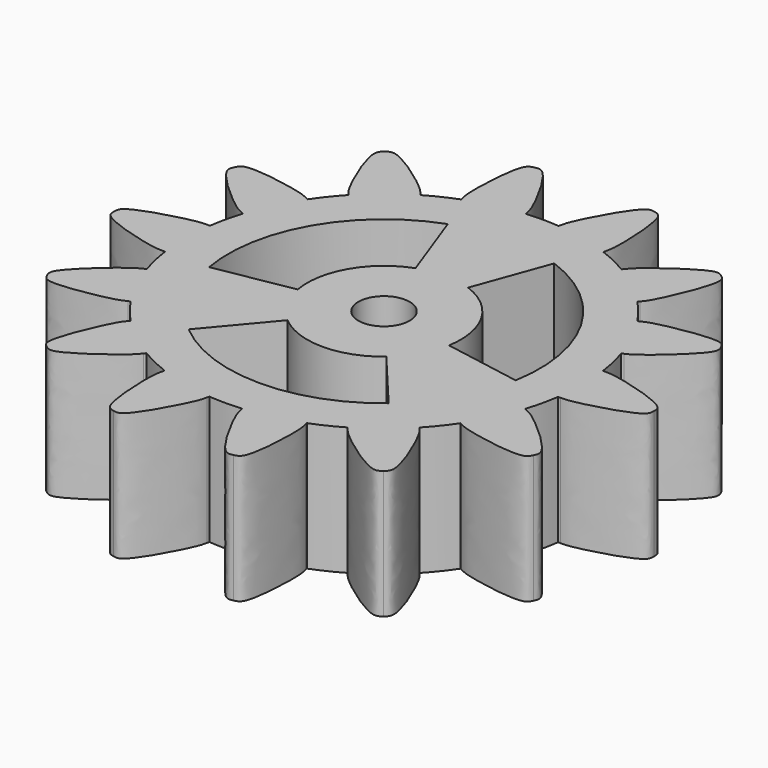
from build123d import *

# Parameters (mm, degrees)
F0_R     = 5.3351790251
F1_DEPTH = 10
F2_DEPTH = 10
F3_COUNT = 14
F4_R     = 15.5
F5_DEPTH = 10
F8_DEPTH = 10
F7_R     = 2
F9_DEPTH = 10


# Not quite as in the source:
# - a feature names something its author has since deleted; it is built from what else it names


with BuildPart() as f1:
    # F0 (on Top) → F1 (new body)
    with BuildSketch(Plane.XY):
        Circle(F0_R)
    extrude(amount=F1_DEPTH)



with BuildPart() as f2:
    # F0 (on Top) → F2 (new body)
    with BuildSketch(Plane.XY):
        with BuildLine():
            Line((-21.0813645951, 0), (-15.5169374102, 0))
            Line((-15.5169374102, 0), (-15.5169374102, 2.1929510403))
            add(Edge.make_bspline(
                [(-15.5169374102, 2.1929510403), (-15.7431787684, 2.1963284468), (-16.4584927159, 2.2070069607), (-21.1021855068, 0.9410331304), (-21.0859014535, 0.2050513008), (-21.0813645951, 0)],
                knots=[0, 0, 0, 0, 0.2502118821, 0.7911020914, 1, 1, 1, 1], degree=3))
        make_face()
        Polygon((-15.5169374102, -2.1929510403), (-13.8607590251, -2.1929510403), (-13.8607590251, 2.1929510403), (-15.5169374102, 2.1929510403), (-15.5169374102, 0), align=None)
        with BuildLine():
            add(Edge.make_bspline(
                [(-15.5169374102, -2.1929510403), (-15.7431787684, -2.1963284468), (-16.4584927159, -2.2070069607), (-21.1021855068, -0.9410331304), (-21.0859014535, -0.2050513008), (-21.0813645951, 0)],
                knots=[0, 0, 0, 0, 0.2502118821, 0.7911020914, 1, 1, 1, 1], degree=3))
            Line((-15.5169374102, -2.1929510403), (-15.5169374102, 0))
            Line((-15.5169374102, 0), (-21.0813645951, 0))
        make_face()
    extrude(amount=F2_DEPTH)


with BuildPart() as f3_1:
    # F3: instance of F2
    add(f2.part.rotate(Axis((0, 0, 10), (0, 0, 1)), 1 * 360 / F3_COUNT))


with BuildPart() as f3_2:
    # F3: instance of F2
    add(f2.part.rotate(Axis((0, 0, 10), (0, 0, 1)), 2 * 360 / F3_COUNT))


with BuildPart() as f3_3:
    # F3: instance of F2
    add(f2.part.rotate(Axis((0, 0, 10), (0, 0, 1)), 3 * 360 / F3_COUNT))


with BuildPart() as f3_4:
    # F3: instance of F2
    add(f2.part.rotate(Axis((0, 0, 10), (0, 0, 1)), 4 * 360 / F3_COUNT))


with BuildPart() as f3_5:
    # F3: instance of F2
    add(f2.part.rotate(Axis((0, 0, 10), (0, 0, 1)), 5 * 360 / F3_COUNT))


with BuildPart() as f3_6:
    # F3: instance of F2
    add(f2.part.rotate(Axis((0, 0, 10), (0, 0, 1)), 6 * 360 / F3_COUNT))


with BuildPart() as f3_7:
    # F3: instance of F2
    add(f2.part.rotate(Axis((0, 0, 10), (0, 0, 1)), 7 * 360 / F3_COUNT))


with BuildPart() as f3_8:
    # F3: instance of F2
    add(f2.part.rotate(Axis((0, 0, 10), (0, 0, 1)), 8 * 360 / F3_COUNT))


with BuildPart() as f3_9:
    # F3: instance of F2
    add(f2.part.rotate(Axis((0, 0, 10), (0, 0, 1)), 9 * 360 / F3_COUNT))


with BuildPart() as f3_10:
    # F3: instance of F2
    add(f2.part.rotate(Axis((0, 0, 10), (0, 0, 1)), 10 * 360 / F3_COUNT))


with BuildPart() as f3_11:
    # F3: instance of F2
    add(f2.part.rotate(Axis((0, 0, 10), (0, 0, 1)), 11 * 360 / F3_COUNT))


with BuildPart() as f3_12:
    # F3: instance of F2
    add(f2.part.rotate(Axis((0, 0, 10), (0, 0, 1)), 12 * 360 / F3_COUNT))


with BuildPart() as f3_13:
    # F3: instance of F2
    add(f2.part.rotate(Axis((0, 0, 10), (0, 0, 1)), 13 * 360 / F3_COUNT))


with BuildPart() as f1_1:
    add(f1.part)

    add(f2.part)  # F5 merges F2

    add(f3_1.part)  # F5 merges F3_1

    add(f3_2.part)  # F5 merges F3_2

    add(f3_3.part)  # F5 merges F3_3

    add(f3_4.part)  # F5 merges F3_4

    add(f3_5.part)  # F5 merges F3_5

    add(f3_6.part)  # F5 merges F3_6

    add(f3_7.part)  # F5 merges F3_7

    add(f3_8.part)  # F5 merges F3_8

    add(f3_9.part)  # F5 merges F3_9

    add(f3_10.part)  # F5 merges F3_10

    add(f3_11.part)  # F5 merges F3_11

    add(f3_12.part)  # F5 merges F3_12

    add(f3_13.part)  # F5 merges F3_13
    # F4 (on Top) → F5 (join)
    with BuildSketch(Plane.XY):
        Circle(F4_R)
    extrude(amount=F5_DEPTH)

    # F6 (on face) → F8 (cut, through all)
    with BuildSketch(Plane.XY.offset(10)):
        with BuildLine():
            ThreePointArc((-5.9088465181, -1.041889066), (-5.1961524227, 3), (-2.05212086, 5.6381557247))
            Line((-2.05212086, 5.6381557247), (-4.1564424219, 11.4197316993))
            ThreePointArc((-4.1564424219, 11.4197316993), (-10.5244816627, 6.076312321), (-11.967998967, -2.110281123))
            Line((-11.967998967, -2.110281123), (-5.9088465181, -1.041889066))
        make_face()
        with BuildLine():
            Line((-3.8567256581, -4.5962666587), (-7.8115565451, -9.3094505764))
            ThreePointArc((-7.8115565451, -9.3094505764), (0, -12.1526246421), (7.8115565451, -9.3094505764))
            Line((7.8115565451, -9.3094505764), (3.8567256581, -4.5962666587))
            ThreePointArc((3.8567256581, -4.5962666587), (0, -6), (-3.8567256581, -4.5962666587))
        make_face()
        with BuildLine():
            ThreePointArc((2.05212086, 5.6381557247), (5.1961524227, 3), (5.9088465181, -1.041889066))
            Line((5.9088465181, -1.041889066), (11.967998967, -2.110281123))
            ThreePointArc((11.967998967, -2.110281123), (10.5244816627, 6.076312321), (4.1564424219, 11.4197316993))
            Line((4.1564424219, 11.4197316993), (2.05212086, 5.6381557247))
        make_face()
    extrude(amount=-F8_DEPTH, mode=Mode.SUBTRACT)

    # F7 (on face) → F9 (cut, through all)
    with BuildSketch(Plane.XY.offset(10)):
        Circle(F7_R)
    extrude(amount=-F9_DEPTH, mode=Mode.SUBTRACT)


solid = f1_1.part
